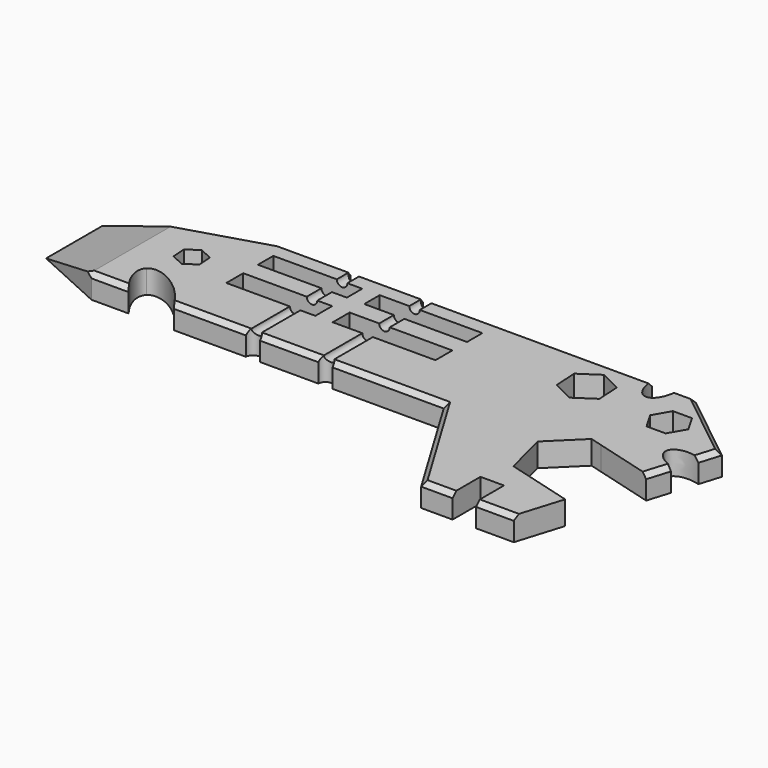
from build123d import *

# Parameters (mm, degrees)
F0_W     = 18.8970365295
F0_H     = 4.4807404547
F0_H_2   = 4.0911118204
F0_W_2   = 21.8192593221
F1_DEPTH = 5
F2_SIZE2 = 14.99999
F2_SIZE  = 4.99999
F3_SIZE  = 1
F4_SIZE2 = 4.99999
F4_SIZE  = 4.99999
F6_DEPTH = 27.7613706845
F8_DEPTH = 25


# Not quite as in the source:
# - a fillet or chamfer is up to 0.001 mm smaller than in the source, because OpenCascade refuses the exact size


with BuildPart() as f1:
    # F0 (on Top) → F1 (new body)
    with BuildSketch(Plane.XY):
        with BuildLine():
            Line((-16.8903698926, 27.7603705845), (-45.5866689581, 27.7603705845))
            Line((-45.5866689581, 27.7603705845), (-64.873334122, 21.915925892))
            Line((-64.873334122, 21.915925892), (-64.873334122, 6.915925892))
            Line((-64.873334122, 6.915925892), (-49.6777754219, 0))
            Line((-49.6777754219, 0), (-34.0925943368, 0))
            Line((-34.0925943368, 0), (-19.6762964765, 0))
            Line((-19.6762964765, 0), (-16.8903698926, 0))
            ThreePointArc((-16.8903698926, 0), (-15.3903698926, 1.5), (-13.8903698926, 0))
            Line((-13.8903698926, 0), (-1.5, 0))
            ThreePointArc((-1.5, 0), (0, 1.5), (1.5, 0))
            Line((1.5, 0), (25.1311098563, 0))
            Line((25.1311098563, 0), (39.7422224801, -24.2544434202))
            Line((39.7422224801, -24.2544434202), (46.4185207422, -24.2544434202))
            Line((46.4185207422, -24.2544434202), (46.4185207422, -20.358148149))
            Line((46.4185207422, -20.358148149), (46.4185207422, -16.8514806193))
            Line((46.4185207422, -16.8514806193), (49.7303717228, -16.8514806193))
            Line((49.7303717228, -16.8514806193), (51.4185207422, -16.8514806193))
            Line((51.4185207422, -16.8514806193), (51.4185207422, -20.358148149))
            Line((51.4185207422, -20.358148149), (51.4185207422, -24.2544434202))
            Line((51.4185207422, -24.2544434202), (59.4185207422, -24.2544434202))
            Line((59.4185207422, -24.2544434202), (62.452050939, -14.383433128))
            Line((62.452050939, -14.383433128), (49.4044023742, -10.7632835876))
            Line((49.4044023742, -10.7632835876), (48.3249483747, -10.4637825028))
            Line((48.3249483747, -10.4637825028), (45.8877734478, -1.0351754323))
            Line((45.8877734478, -1.0351754323), (52.3168499865, 5.2811170366))
            Line((52.3168499865, 5.2811170366), (54.9051102333, 4.5629884715))
            Line((54.9051102333, 4.5629884715), (67.2241984802, 1.1449824274))
            Line((67.2241984802, 1.1449824274), (68.6868362688, 5.9043590378))
            add(Edge.make_bspline(
                [(70.3025076165, 11.1617019577), (65.5215596777, 12.625438507), (64.7137240038, 9.9967670471), (63.90588833, 7.3680955871), (68.6868362688, 5.9043590378)],
                knots=[1.569962617, 1.569962617, 1.569962617, 3.1407589438, 3.1407589438, 4.7115552706, 4.7115552706, 4.7115552706], degree=2, weights=[1, 0.7071067812, 1, 0.7071067812, 1]))
            Line((70.3025076165, 11.1617019577), (71.6918544178, 15.6825920379))
            Line((71.6918544178, 15.6825920379), (56.4962957177, 27.7603705845))
            Line((56.4962957177, 27.7603705845), (52.6956264079, 27.7603705845))
            add(Edge.make_bspline(
                [(47.1956264079, 27.7603705845), (47.1956264079, 22.7603705845), (49.9456264079, 22.7603705845), (52.6956264079, 22.7603705845), (52.6956264079, 27.7603705845)],
                knots=[4.7123889804, 4.7123889804, 4.7123889804, 6.2831853072, 6.2831853072, 7.853981634, 7.853981634, 7.853981634], degree=2, weights=[1, 0.7071067812, 1, 0.7071067812, 1]))
            Line((47.1956264079, 27.7603705845), (1.5, 27.7603705845))
            ThreePointArc((1.5, 27.7603705845), (0, 26.2603705845), (-1.5, 27.7603705845))
            Line((-1.5, 27.7603705845), (-13.8903698926, 27.7603705845))
            ThreePointArc((-13.8903698926, 27.7603705845), (-15.3903698926, 26.2603705845), (-16.8903698926, 27.7603705845))
        make_face()
        with Locations((-20.5529624662, 13.4422218106)):
            Rectangle(F0_W, F0_H, mode=Mode.SUBTRACT)
        Polygon((-37.830516684, 16.5674356593), (-37.6374373089, 13.573655381), (-40.1335873958, 11.9095535981), (-42.8228168577, 13.2392320936), (-43.0158962327, 16.2330123719), (-40.5197461458, 17.8971141548), align=None, mode=Mode.SUBTRACT)
        with Locations((-20.5529624662, 21.6244432194)):
            Rectangle(F0_W, F0_H_2, mode=Mode.SUBTRACT)
        with Locations((3.5066673065, 13.4422218106)):
            Rectangle(F0_W_2, F0_H, mode=Mode.SUBTRACT)
        with Locations((3.5066673065, 21.6244432194)):
            Rectangle(F0_W_2, F0_H_2, mode=Mode.SUBTRACT)
        Polygon((44.0257825333, 22.3436092413), (44.3475814916, 17.3539754441), (40.1873313468, 14.5804724726), (35.7052822437, 16.7966032984), (35.3834832853, 21.7862370956), (39.5437334301, 24.5597400671), align=None, mode=Mode.SUBTRACT)
        Polygon((62.6884105106, 18.0203692007), (60.6638360993, 14.5137034565), (56.6146872766, 14.5137034565), (54.5901128653, 18.0203692007), (56.6146872766, 21.5270349448), (60.6638360993, 21.5270349448), align=None, mode=Mode.SUBTRACT)
    extrude(amount=F1_DEPTH)

    # F2 (size 5 and 15 in the source; OpenCascade refuses exactly that, so slightly less here)
    f2_edges = [f1.edges().sort_by_distance(p)[0] for p in [
        (-64.873334, 14.415926, 5),
    ]]
    f2_side = f1.faces().sort_by_distance((-64.873334, 14.415926, 2.5))[0]
    chamfer(f2_edges, length=F2_SIZE, length2=F2_SIZE2, reference=f2_side)

    # F3
    f3_edges = [f1.edges().sort_by_distance(p)[0] for p in [
        (13.315555, 0, 5),
        (-7.695185, 0, 5),
        (-7.695185, 27.760371, 5),
        (24.347813, 27.760371, 5),
        (-31.238519, 27.760371, 5),
        (32.436666, -12.127222, 5),
        (67.955517, 3.524671, 5),
        (64.094075, 21.721481, 5),
        (70.997181, 13.422147, 5),
        (54.595961, 27.760371, 5),
        (55.418521, -24.254443, 5),
        (43.080372, -24.254443, 5),
        (-33.284073, 0, 5),
    ]]
    chamfer(f3_edges, length=F3_SIZE)

    # F4 (size 5 and 5 in the source; OpenCascade refuses exactly that, so slightly less here)
    f4_edges = [f1.edges().sort_by_distance(p)[0] for p in [
        (-49.380006, 26.610874, 5),
    ]]
    chamfer(f4_edges, length=F4_SIZE, length2=F4_SIZE2)

    # F5 (on face) → F6 (cut, through all)
    with BuildSketch(Plane.XZ):
        with BuildLine():
            ThreePointArc((-16.5084038813, 5), (-15.3903698926, 3.8819660113), (-14.2723359038, 5))
            Line((-14.2723359038, 5), (-16.5084038813, 5))
        make_face()
        with BuildLine():
            Line((-16.5084038813, 5), (-14.2723359038, 5))
            ThreePointArc((-14.2723359038, 5), (-15.3903698926, 6.1180339887), (-16.5084038813, 5))
        make_face()
        with BuildLine():
            ThreePointArc((-1.1180339887, 5), (0, 3.8819660113), (1.1180339887, 5))
            Line((1.1180339887, 5), (-1.1180339887, 5))
        make_face()
        with BuildLine():
            Line((-1.1180339887, 5), (1.1180339887, 5))
            ThreePointArc((1.1180339887, 5), (0, 6.1180339887), (-1.1180339887, 5))
        make_face()
    extrude(amount=-F6_DEPTH, mode=Mode.SUBTRACT)

    # F7 (on face) → F8 (cut)
    with BuildSketch(Plane.XY.offset(5)):
        with BuildLine():
            add(Edge.make_bspline(
                [(-43.646056205, 7.0345965214), (-48.3034396963, 2.4297517681), (-37.0249652513, -4.3197206373), (-25.7464908063, -11.0691930428), (-32.36758176, 0.2851241159), (-38.9886727137, 11.6394412747), (-43.646056205, 7.0345965214)],
                knots=[0, 0, 0, 2.0943951024, 2.0943951024, 4.1887902048, 4.1887902048, 6.2831853072, 6.2831853072, 6.2831853072], degree=2, weights=[1, 0.5, 1, 0.5, 1, 0.5, 1]))
        make_face()
    extrude(amount=-F8_DEPTH, mode=Mode.SUBTRACT)


solid = f1.part
